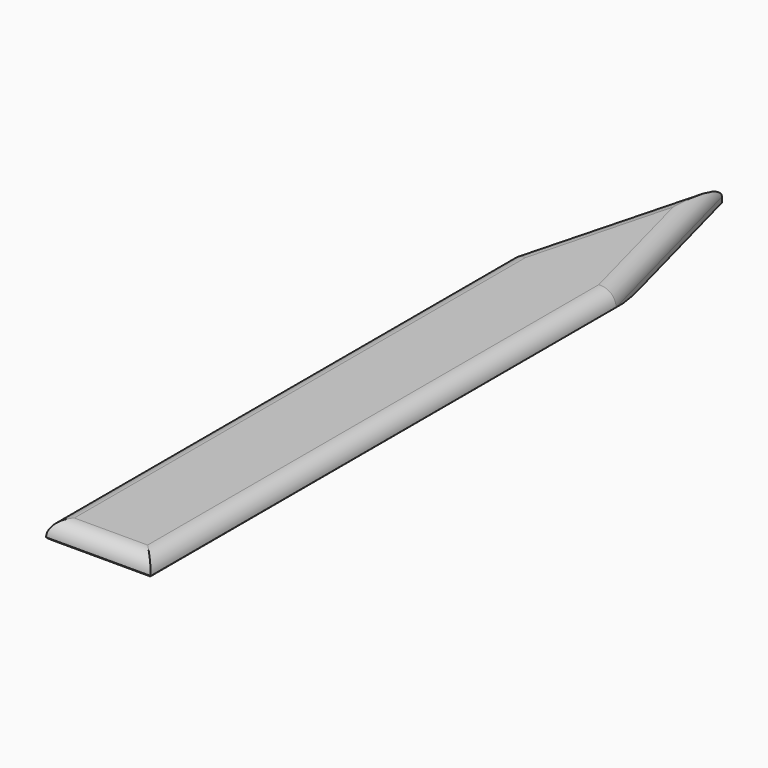
from build123d import *

# Parameters (mm, degrees)
F0_W        = 12.7
F0_H        = 94.5614505536
F1_DEPTH    = 2.54
F3_DEPTH    = 3.81
F4_R        = 1.905
F5_T1_DEPTH = 19.7995158286
F5_T3_DEPTH = 80.155505846


# Not quite as in the source:
# - a fillet or chamfer that OpenCascade refuses, or shapes differently, is made with other operations: its cross-section is extruded or revolved along the edge and cut away or added


with BuildPart() as f1:
    # F0 (on Top) → F1 (new body)
    with BuildSketch(Plane.XY):
        with Locations((-6.35, -5.6614459495)):
            Rectangle(F0_W, F0_H)
    extrude(amount=F1_DEPTH)

    # F2 (on face) → F3 (cut)
    with BuildSketch(Plane.XY.offset(2.54)):
        Polygon((-12.7, 17.6289882511), (-6.35, 41.6192793273), (-12.7, 41.6192793273), align=None)
        Polygon((0, 41.6192793273), (-6.35, 41.6192793273), (0, 17.6289882511), align=None)
    extrude(amount=-F3_DEPTH, mode=Mode.SUBTRACT)

    # F4
    f4_edges = [f1.edges().sort_by_distance(p)[0] for p in [
        (-3.175, 29.624134, 2.54),
        (-12.7, -17.656591, 2.54),
        (0, -17.656591, 2.54),
        (-6.35, -52.942171, 2.54),
        (-9.525, 29.624134, 2.54),
    ]]
    fillet(f4_edges, radius=F4_R)

    # F5: fillet of radius 1.905 on 3 edges, made by hand

    # F5_s2 → F5_t1 (cut)
    with BuildSketch(Plane.YZ.offset(-16.2497579143)):
        with BuildLine():
            ThreePointArc((-51.5222680606, 0), (-52.299981054, 0.1659808799), (-52.9421712264, 0.635))
            Line((-52.9421712264, 0.635), (-52.9421712264, 0))
            Line((-52.9421712264, 0), (-51.5222680606, 0))
        make_face()
    extrude(amount=F5_T1_DEPTH, mode=Mode.SUBTRACT)

    # F5_s4 → F5_t3 (cut)
    with BuildSketch(Plane.XZ.offset(-23.6635767054)):
        with BuildLine():
            ThreePointArc((-11.2800968343, 0), (-12.0578098276, 0.1659808799), (-12.7, 0.635))
            Line((-12.7, 0.635), (-12.7, 0))
            Line((-12.7, 0), (-11.2800968343, 0))
        make_face()
        with BuildLine():
            ThreePointArc((-1.4199031657, 0), (-0.6421901724, 0.1659808799), (0, 0.635))
            Line((0, 0.635), (0, 0))
            Line((0, 0), (-1.4199031657, 0))
        make_face()
    extrude(amount=F5_T3_DEPTH, mode=Mode.SUBTRACT)


solid = f1.part
